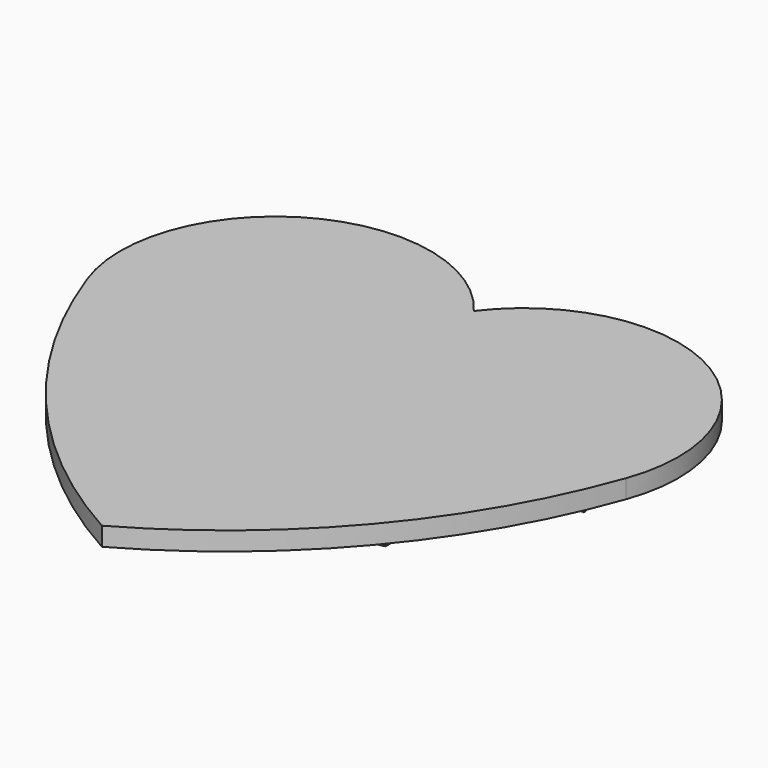
from build123d import *

# Parameters (mm, degrees)
F1_DEPTH     = 3
F2_TEXT_SIZE = 10.0384290879
F3_DEPTH     = 5


# Not quite as in the source:
# - Text() gives the source's letters only with a copy of the font that has no kerning and outlines rounded to 1/6400 em; it was checked with that copy


with BuildPart() as f1:
    # F0 (on Top) → F1 (new body)
    with BuildSketch(Plane.XY):
        with BuildLine():
            ThreePointArc((0, 25), (-31.9332419898, 31.9681072379), (-43.4694905862, 1.387043967))
            ThreePointArc((-43.4694905862, 1.387043967), (-26.3959328799, -28.2494845467), (0, -50))
            ThreePointArc((0, -50), (26.3959328799, -28.2494845467), (43.4694905862, 1.387043967))
            ThreePointArc((43.4694905862, 1.387043967), (31.9332419898, 31.9681072379), (0, 25))
        make_face()
    extrude(amount=-F1_DEPTH)

    # F2 (on face) → F3 (join)
    with BuildSketch(Plane(origin=(0, 0, -3), x_dir=(1, 0, 0), z_dir=(0, 0, -1))):
        with Locations(Location((37.4198129298, -2.7723310567), (0, 0, -180))):
            Text('YOU MAKE ME', F2_TEXT_SIZE, font='Tinos', font_style=FontStyle.BOLD, text_align=(TextAlign.LEFT, TextAlign.BOTTOM))
        with Locations(Location((27.3813838418, 8.7718623944), (0, 0, -180))):
            Text('FEEL LIKE', F2_TEXT_SIZE, font='Tinos', font_style=FontStyle.BOLD, text_align=(TextAlign.LEFT, TextAlign.BOTTOM))
        with Locations(Location((22.3621692979, 20.3160558455), (0, 0, -180))):
            Text('SMILING', F2_TEXT_SIZE, font='Tinos', font_style=FontStyle.BOLD, text_align=(TextAlign.LEFT, TextAlign.BOTTOM))
    extrude(amount=F3_DEPTH)


solid = f1.part
